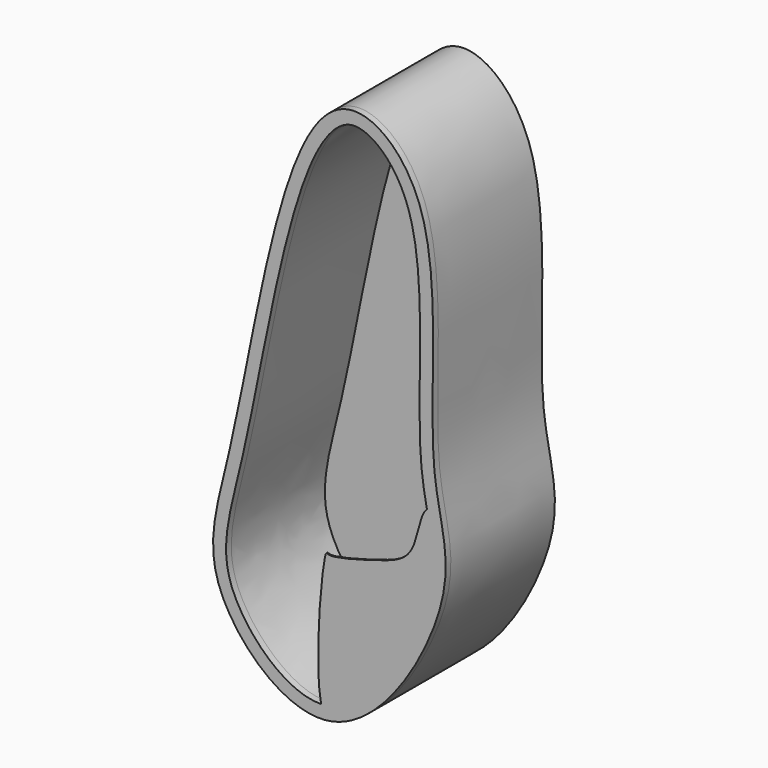
from build123d import *

# Parameters (mm, degrees)
F1_DEPTH = 25.4
F2_DEPTH = 1.27
F3_T     = -2.54
F5_DEPTH = 0.254


with BuildPart() as f1:
    # F0 (on Front) → F1 (new body)
    with BuildSketch(Plane.XZ):
        with BuildLine():
            add(Edge.make_bspline(
                [(-28.9597790688, 11.8837589398), (-31.4377866608, 1.2277911003), (-36.4460675325, -12.5378963169), (-7.1190911595, -40.4883894763), (17.7822904419, 1.9642091519), (7.985630494, 20.070756183), (14.1815873575, 66.3556960204), (-5.5131674944, 82.4294765137), (-19.6316564772, 65.0365760226), (-25.2947068068, 27.64436124), (-28.9597790688, 11.8837589398)],
                knots=[0, 0, 0, 0, 0.1164380641, 0.2350145668, 0.3739432864, 0.482027521, 0.6360847726, 0.7333686026, 0.8277834498, 1, 1, 1, 1], degree=3))
        make_face()
    extrude(amount=F1_DEPTH)

    # F2 (add): a face of the model
    f2_faces = [f1.faces().sort_by_distance(p)[0] for p in [
        (-7.9018551825, -25.4, 20.8918797423),
    ]]
    extrude(f2_faces, amount=F2_DEPTH)

    # F3
    f3_openings = [f1.faces().sort_by_distance(p)[0] for p in [
        (-7.901855, -26.67, 20.89188),
    ]]
    offset(amount=F3_T, openings=f3_openings)

    # F4 (on face) → F5 (join)
    with BuildSketch(Plane.XZ.offset(26.67)):
        with BuildLine():
            add(Edge.make_bspline(
                [(-11.1047399491, -26.1826142582), (-12.5666481764, -19.2337451121), (-10.6688882782, 1.2355031782), (-9.5059025927, -0.6244537334), (0.7209441111, 2.2842610441), (7.6527554831, 4.6463133934), (8.2235539673, 13.0724580126), (9.5720154365, 13.9826734446)],
                knots=[0.0250811952, 0.0250811952, 0.0250811952, 0.0250811952, 0.1723913176, 0.1948681832, 0.2962096699, 0.3864378573, 0.4786527042, 0.4786527042, 0.4786527042, 0.4786527042], degree=3))
            add(Edge.make_bspline(
                [(9.5720154365, 13.9826734446), (9.6385221448, 13.6358396064), (9.7053451031, 13.2890659815), (9.7721915849, 12.9422951284), (9.8387421398, 12.595466219), (9.9046505055, 12.2485150212), (9.9695453328, 11.9013742278), (10.033033721, 11.5539741328), (10.1942284745, 10.6451085245), (10.289017333, 10.083145259), (10.3773542535, 9.5200563659), (10.457400857, 8.955646553), (10.5272572626, 8.3898300276), (10.5851241218, 7.8226508616), (10.6294831308, 7.2543065975), (10.6813288218, 6.2617004469), (10.6953476697, 5.8377863658), (10.7007998023, 5.4136181328), (10.697347206, 4.989399869), (10.6847946673, 4.5653452033), (10.6630891207, 4.1416777653), (10.632304726, 3.7186316784), (10.5728339575, 3.0860622134), (10.5506552829, 2.8738959031), (10.5260119135, 2.6598452326), (10.4988366055, 2.44380393), (10.469060609, 2.2256673409), (10.4366136679, 2.0053324282), (10.4014240202, 1.7826977724), (10.321158452, 1.3074391946), (10.275472689, 1.0546394283), (10.2262617813, 0.7987470847), (10.1733083336, 0.5394201414), (10.1164636731, 0.2764544569), (10.0557154405, 0.0097713747), (9.9911359783, -0.2605697819), (9.7738423919, -1.1299559709), (9.6117191777, -1.722224916), (9.4377780297, -2.3112114899), (9.2530355766, -2.896915842), (9.0582781979, -3.4793255967), (8.8541306652, -4.0584372519), (8.6410733823, -4.6342616361), (8.1732409262, -5.8430736417), (7.9164880172, -6.4752285656), (7.6497480916, -7.1032954751), (7.373415648, -7.7272270969), (7.0877837177, -8.3469464023), (6.7930654253, -8.9623559735), (6.489403713, -9.5733422559), (5.7413526989, -11.0248377795), (5.288652241, -11.8609700665), (4.8189541936, -12.68785226), (4.3322439878, -13.5049728295), (3.8283425487, -14.3116496767), (3.3069049824, -15.1070282653), (2.7673815497, -15.8900562171), (1.6849990428, -17.3812827195), (1.1445724004, -18.0908853481), (0.5868758904, -18.7873333134), (0.011062951, -19.4692853586), (-0.5838198943, -20.1349209288), (-1.1988532544, -20.7819217662), (-1.8353608472, -21.4073666954), (-3.0854570243, -22.5441309854), (-3.6934961237, -23.0597324209), (-4.3213694383, -23.5522616366), (-4.9706400424, -24.0182132872), (-5.6424283169, -24.4525209256), (-6.3374005003, -24.8485633231), (-7.0558729767, -25.1979873283), (-7.9322570295, -25.5429107473), (-8.0659826965, -25.593366596), (-8.1993259361, -25.6414985239), (-8.3322742867, -25.6873037697), (-8.4648175109, -25.7307806798), (-8.5969475956, -25.7719287089), (-8.7286587519, -25.8107484197), (-9.0792241283, -25.9081917493), (-9.2965267639, -25.9623941299), (-9.5123352225, -26.0102385876), (-9.7272610712, -26.0516619892), (-9.941936721, -26.0866908013), (-10.156970989, -26.115615641), (-10.3729710471, -26.1387976793), (-10.654644848, -26.1611975714), (-10.7187276452, -26.1657773724), (-10.7828805874, -26.1698479529), (-10.8471050012, -26.1734108713), (-10.9114021001, -26.1764676012), (-10.9757729848, -26.1790195379), (-11.0402186428, -26.1810680043), (-11.1047399491, -26.1826142582)],
                knots=[0.6203608595, 0.6203608595, 0.6203608595, 0.6203608595, 0.6203608595, 0.6203608595, 0.6203608595, 0.6203608595, 0.6203608595, 0.6324591526, 0.6324591526, 0.6324591526, 0.6324591526, 0.6324591526, 0.6324591526, 0.6324591526, 0.6519822536, 0.6519822536, 0.6519822536, 0.6519822536, 0.6519822536, 0.6519822536, 0.6519822536, 0.6665082529, 0.6665082529, 0.6665082529, 0.6665082529, 0.6665082529, 0.6665082529, 0.6665082529, 0.6737471684, 0.6737471684, 0.6737471684, 0.6737471684, 0.6737471684, 0.6737471684, 0.6737471684, 0.6817964032, 0.6817964032, 0.6817964032, 0.6817964032, 0.6817964032, 0.6817964032, 0.6817964032, 0.6993088919, 0.6993088919, 0.6993088919, 0.6993088919, 0.6993088919, 0.6993088919, 0.6993088919, 0.7187687014, 0.7187687014, 0.7187687014, 0.7187687014, 0.7187687014, 0.7187687014, 0.7187687014, 0.7458859291, 0.7458859291, 0.7458859291, 0.7458859291, 0.7458859291, 0.7458859291, 0.7458859291, 0.7713279381, 0.7713279381, 0.7713279381, 0.7713279381, 0.7713279381, 0.7713279381, 0.7713279381, 0.7940839213, 0.7940839213, 0.7940839213, 0.7940839213, 0.7940839213, 0.7940839213, 0.7940839213, 0.7981947468, 0.7981947468, 0.7981947468, 0.7981947468, 0.7981947468, 0.7981947468, 0.7981947468, 0.8050605972, 0.8050605972, 0.8050605972, 0.8050605972, 0.8050605972, 0.8050605972, 0.8050605972, 0.8070798555, 0.8070798555, 0.8070798555, 0.8070798555, 0.8070798555, 0.8070798555, 0.8070798555, 0.8070798555, 0.8070798555], degree=8))
        make_face()
    extrude(amount=-F5_DEPTH)


solid = f1.part
